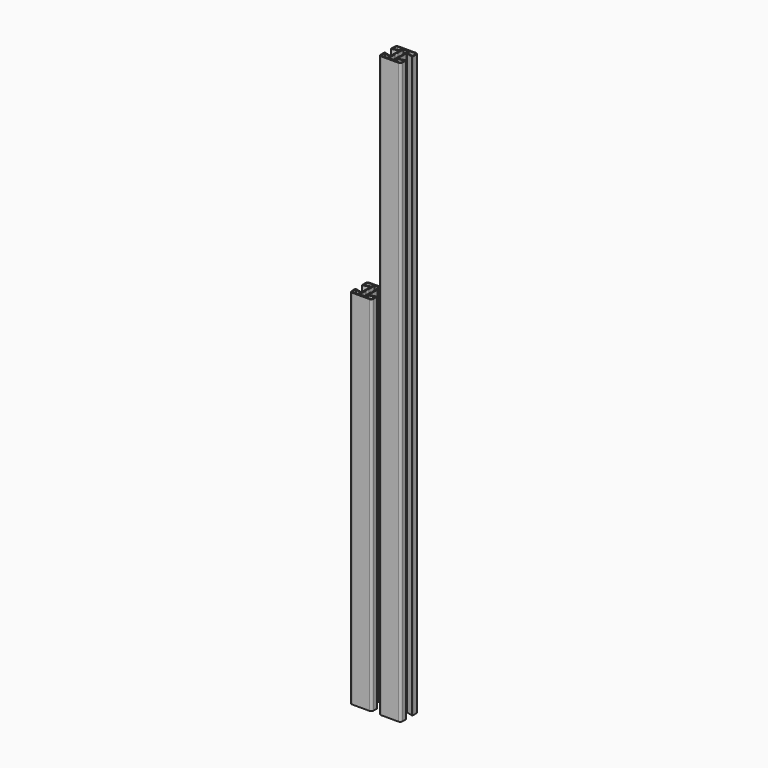
from build123d import *

# Parameters (mm, degrees)
F1_DEPTH = 1000
F2_DEPTH = 1600


# Not quite as in the source:
# - ends of sketch curves that miss each other by under 0.0002 mm in the source are joined


with BuildPart() as f1:
    # F0 (on Top) → F1 (new body)
    with BuildSketch(Plane.XY):
        with BuildLine():
            ThreePointArc((11.2588189596, -15.2716838492), (10.3912385359, -15.0991113133), (10, -14.305758))
            Line((10, -14.305758), (10, 14.305758))
            ThreePointArc((10, 14.305758), (10.3912385359, 15.0991113133), (11.2588189596, 15.2716838492))
            Line((11.2588189596, 15.2716838492), (28.426476, 10.671624))
            ThreePointArc((28.426476, 10.671624), (29.5109517857, 10.8873403242), (30, 11.879032))
            Line((30, 11.879032), (30, 24))
            ThreePointArc((30, 24), (28.2426406871, 28.2426406871), (24, 30))
            Line((24, 30), (-24, 30))
            ThreePointArc((-24, 30), (-28.2426406871, 28.2426406871), (-30, 24))
            Line((-30, 24), (-30, 11.879032))
            ThreePointArc((-30, 11.879032), (-29.5109517857, 10.8873403242), (-28.4264761923, 10.6716247175))
            Line((-28.4264761923, 10.6716247175), (-11.258819, 15.271684))
            ThreePointArc((-11.258819, 15.271684), (-10.3912385359, 15.0991113133), (-10, 14.305758))
            Line((-10, 14.305758), (-10, -14.305758))
            ThreePointArc((-10, -14.305758), (-10.3912385359, -15.0991113133), (-11.2588189596, -15.2716838492))
            Line((-11.2588189596, -15.2716838492), (-28.426476, -10.671624))
            ThreePointArc((-28.426476, -10.671624), (-29.5109517857, -10.8873403242), (-30, -11.879032))
            Line((-30, -11.879032), (-30, -24))
            ThreePointArc((-30, -24), (-28.2426406871, -28.2426406871), (-24, -30))
            Line((-24, -30), (24, -30))
            ThreePointArc((24, -30), (28.2426406871, -28.2426406871), (30, -24))
            Line((30, -24), (30, -11.879032))
            ThreePointArc((30, -11.879032), (29.5109517857, -10.8873403242), (28.4264761923, -10.6716247175))
            Line((28.4264761923, -10.6716247175), (11.2588189596, -15.2716838492))
        make_face()
        with BuildLine():
            Line((-11, -27.25), (-24, -27.25))
            ThreePointArc((-24, -27.25), (-26.2980970389, -26.2980970389), (-27.25, -24))
            Line((-27.25, -24), (-27.25, -15.137095))
            ThreePointArc((-27.25, -15.137095), (-26.8587614641, -14.3437416867), (-25.9911810404, -14.1711691508))
            Line((-25.9911810404, -14.1711691508), (-10.741181, -18.257395))
            ThreePointArc((-10.741181, -18.257395), (-10.2066466079, -18.6145586385), (-10, -19.22332))
            Line((-10, -19.22332), (-10, -26.25))
            ThreePointArc((-10, -26.25), (-10.2928932188, -26.9571067812), (-11, -27.25))
        make_face(mode=Mode.SUBTRACT)
        with BuildLine():
            Line((10.741181, -18.257395), (25.991181, -14.171169))
            ThreePointArc((25.991181, -14.171169), (26.8587614641, -14.3437416867), (27.25, -15.137095))
            Line((27.25, -15.137095), (27.25, -24))
            ThreePointArc((27.25, -24), (26.2980970389, -26.2980970389), (24, -27.25))
            Line((24, -27.25), (11, -27.25))
            ThreePointArc((11, -27.25), (10.2928932188, -26.9571067812), (10, -26.25))
            Line((10, -26.25), (10, -19.22332))
            ThreePointArc((10, -19.22332), (10.2066466079, -18.6145586385), (10.741181, -18.257395))
        make_face(mode=Mode.SUBTRACT)
        with BuildLine():
            Line((5.2, -25.2), (-5.2, -25.2))
            ThreePointArc((-5.2, -25.2), (-5.9071067812, -24.9071067812), (-6.2, -24.2))
            Line((-6.2, -24.2), (-6.2, -5.4))
            ThreePointArc((-6.2, -5.4), (-6.2513167019, -5.083772234), (-6.4, -4.8))
            ThreePointArc((-6.4, -4.8), (-8, 0), (-6.4, 4.8))
            ThreePointArc((-6.4, 4.8), (-6.2513167019, 5.083772234), (-6.2, 5.4))
            Line((-6.2, 5.4), (-6.2, 24.2))
            ThreePointArc((-6.2, 24.2), (-5.9071067812, 24.9071067812), (-5.2, 25.2))
            Line((-5.2, 25.2), (5.2, 25.2))
            ThreePointArc((5.2, 25.2), (5.9071067812, 24.9071067812), (6.2, 24.2))
            Line((6.2, 24.2), (6.2, 5.4))
            ThreePointArc((6.2, 5.4), (6.2513167019, 5.083772234), (6.4, 4.8))
            ThreePointArc((6.4, 4.8), (8, 0), (6.4, -4.8))
            ThreePointArc((6.4, -4.8), (6.2513167019, -5.083772234), (6.2, -5.4))
            Line((6.2, -5.4), (6.2, -24.2))
            ThreePointArc((6.2, -24.2), (5.9071067812, -24.9071067812), (5.2, -25.2))
        make_face(mode=Mode.SUBTRACT)
        with BuildLine():
            Line((-10.741181, 18.257395), (-25.991181, 14.171169))
            ThreePointArc((-25.991181, 14.171169), (-26.8587614641, 14.3437416867), (-27.25, 15.137095))
            Line((-27.25, 15.137095), (-27.25, 24))
            ThreePointArc((-27.25, 24), (-26.2980970389, 26.2980970389), (-24, 27.25))
            Line((-24, 27.25), (-11, 27.25))
            ThreePointArc((-11, 27.25), (-10.2928932188, 26.9571067812), (-10, 26.25))
            Line((-10, 26.25), (-10, 19.22332))
            ThreePointArc((-10, 19.22332), (-10.2066466079, 18.6145586385), (-10.741181, 18.257395))
        make_face(mode=Mode.SUBTRACT)
        with BuildLine():
            Line((11, 27.25), (24, 27.25))
            ThreePointArc((24, 27.25), (26.2980970389, 26.2980970389), (27.25, 24))
            Line((27.25, 24), (27.25, 15.137095))
            ThreePointArc((27.25, 15.137095), (26.8587614641, 14.3437416867), (25.9911810404, 14.1711691508))
            Line((25.9911810404, 14.1711691508), (10.741181, 18.257395))
            ThreePointArc((10.741181, 18.257395), (10.2066466079, 18.6145586385), (10, 19.22332))
            Line((10, 19.22332), (10, 26.25))
            ThreePointArc((10, 26.25), (10.2928932188, 26.9571067812), (11, 27.25))
        make_face(mode=Mode.SUBTRACT)
    extrude(amount=F1_DEPTH)


with BuildPart() as f2:
    # F0 (on Top) → F2 (new body)
    with BuildSketch(Plane.XY):
        with BuildLine():
            ThreePointArc((50, -24), (51.7573593129, -28.2426406871), (56, -30))
            Line((56, -30), (104, -30))
            ThreePointArc((104, -30), (108.2426406871, -28.2426406871), (110, -24))
            Line((110, -24), (110, -11.879032))
            ThreePointArc((110, -11.879032), (109.5109517857, -10.8873403242), (108.4264761923, -10.6716247175))
            Line((108.4264761923, -10.6716247175), (91.258819, -15.271684))
            ThreePointArc((91.258819, -15.271684), (90.3912385359, -15.0991113133), (90, -14.305758))
            Line((90, -14.305758), (90, 14.305758))
            ThreePointArc((90, 14.305758), (90.3912385359, 15.0991113133), (91.2588189596, 15.2716838492))
            Line((91.2588189596, 15.2716838492), (108.426476, 10.671624))
            ThreePointArc((108.426476, 10.671624), (109.5109517857, 10.8873403242), (110, 11.879032))
            Line((110, 11.879032), (110, 24))
            ThreePointArc((110, 24), (108.2426406871, 28.2426406871), (104, 30))
            Line((104, 30), (56, 30))
            ThreePointArc((56, 30), (51.7573593129, 28.2426406871), (50, 24))
            Line((50, 24), (50, 11.879032))
            ThreePointArc((50, 11.879032), (50.4890482143, 10.8873403242), (51.5735238077, 10.6716247175))
            Line((51.5735238077, 10.6716247175), (68.741181, 15.271684))
            ThreePointArc((68.741181, 15.271684), (69.6087614641, 15.0991113133), (70, 14.305758))
            Line((70, 14.305758), (70, -14.305758))
            ThreePointArc((70, -14.305758), (69.6087614641, -15.0991113133), (68.7411810404, -15.2716838492))
            Line((68.7411810404, -15.2716838492), (51.573524, -10.671624))
            ThreePointArc((51.573524, -10.671624), (50.4890482143, -10.8873403242), (50, -11.879032))
            Line((50, -11.879032), (50, -24))
        make_face()
        with BuildLine():
            Line((54.008819, -14.171169), (69.258819, -18.257395))
            ThreePointArc((69.258819, -18.257395), (69.7933533921, -18.6145586385), (70, -19.22332))
            Line((70, -19.22332), (70, -26.25))
            ThreePointArc((70, -26.25), (69.7071067812, -26.9571067812), (69, -27.25))
            Line((69, -27.25), (56, -27.25))
            ThreePointArc((56, -27.25), (53.7019029611, -26.2980970389), (52.75, -24))
            Line((52.75, -24), (52.75, -15.137095))
            ThreePointArc((52.75, -15.137095), (53.1412385359, -14.3437416867), (54.008819, -14.171169))
        make_face(mode=Mode.SUBTRACT)
        with BuildLine():
            Line((104, -27.25), (91, -27.25))
            ThreePointArc((91, -27.25), (90.2928932188, -26.9571067812), (90, -26.25))
            Line((90, -26.25), (90, -19.22332))
            ThreePointArc((90, -19.22332), (90.2066466079, -18.6145586385), (90.7411807904, -18.2573942178))
            Line((90.7411807904, -18.2573942178), (105.991181, -14.171169))
            ThreePointArc((105.991181, -14.171169), (106.8587614641, -14.3437416867), (107.25, -15.137095))
            Line((107.25, -15.137095), (107.25, -24))
            ThreePointArc((107.25, -24), (106.2980970389, -26.2980970389), (104, -27.25))
        make_face(mode=Mode.SUBTRACT)
        with BuildLine():
            Line((86.2, 24.2), (86.2, 5.4))
            ThreePointArc((86.2, 5.4), (86.2513167019, 5.083772234), (86.4, 4.8))
            ThreePointArc((86.4, 4.8), (88, 0), (86.4, -4.8))
            ThreePointArc((86.4, -4.8), (86.2513167019, -5.083772234), (86.2, -5.4))
            Line((86.2, -5.4), (86.2, -24.2))
            ThreePointArc((86.2, -24.2), (85.9071067812, -24.9071067812), (85.2, -25.2))
            Line((85.2, -25.2), (74.8, -25.2))
            ThreePointArc((74.8, -25.2), (74.0928932188, -24.9071067812), (73.8, -24.2))
            Line((73.8, -24.2), (73.8, -5.4))
            ThreePointArc((73.8, -5.4), (73.7486832981, -5.083772234), (73.6, -4.8))
            ThreePointArc((73.6, -4.8), (72, 0), (73.6, 4.8))
            ThreePointArc((73.6, 4.8), (73.7486832981, 5.083772234), (73.8, 5.4))
            Line((73.8, 5.4), (73.8, 24.2))
            ThreePointArc((73.8, 24.2), (74.0928932188, 24.9071067812), (74.8, 25.2))
            Line((74.8, 25.2), (85.2, 25.2))
            ThreePointArc((85.2, 25.2), (85.9071067812, 24.9071067812), (86.2, 24.2))
        make_face(mode=Mode.SUBTRACT)
        with BuildLine():
            Line((69.258819, 18.257395), (54.008819, 14.171169))
            ThreePointArc((54.008819, 14.171169), (53.1412385359, 14.3437416867), (52.75, 15.137095))
            Line((52.75, 15.137095), (52.75, 24))
            ThreePointArc((52.75, 24), (53.7019029611, 26.2980970389), (56, 27.25))
            Line((56, 27.25), (69, 27.25))
            ThreePointArc((69, 27.25), (69.7071067812, 26.9571067812), (70, 26.25))
            Line((70, 26.25), (70, 19.22332))
            ThreePointArc((70, 19.22332), (69.7933533921, 18.6145586385), (69.258819, 18.257395))
        make_face(mode=Mode.SUBTRACT)
        with BuildLine():
            Line((105.991181, 14.171169), (90.741181, 18.257395))
            ThreePointArc((90.741181, 18.257395), (90.2066466079, 18.6145586385), (90, 19.22332))
            Line((90, 19.22332), (90, 26.25))
            ThreePointArc((90, 26.25), (90.2928932188, 26.9571067812), (91, 27.25))
            Line((91, 27.25), (104, 27.25))
            ThreePointArc((104, 27.25), (106.2980970389, 26.2980970389), (107.25, 24))
            Line((107.25, 24), (107.25, 15.137095))
            ThreePointArc((107.25, 15.137095), (106.8587614641, 14.3437416867), (105.991181, 14.171169))
        make_face(mode=Mode.SUBTRACT)
    extrude(amount=F2_DEPTH)


solid = Compound([f1.part, f2.part])
